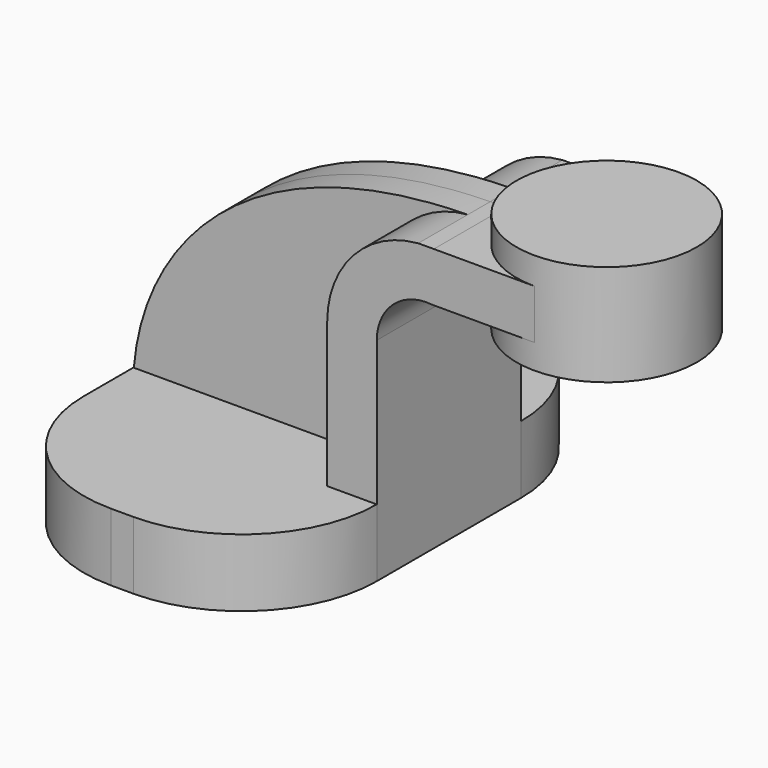
from build123d import *

# Parameters (mm, degrees)
F1_DEPTH = 63.5
F2_DEPTH = 25.4
F3_DEPTH = 7.9375
F5_R     = 38.1


with BuildPart() as f1:
    # F0 (on Front) → F1 (new body, symmetric)
    with BuildSketch(Plane.XZ):
        Polygon((41.275, 9.525), (27.305, 9.525), (-41.1475321427, 9.525), (-41.275, 9.525), (-41.275, -9.525), (41.275, -9.525), align=None)
    extrude(amount=F1_DEPTH, both=True)

    # F0 (on Front) → F2 (join, symmetric)
    with BuildSketch(Plane.XZ):
        with BuildLine():
            Line((27.305, 50.2448773877), (27.305, 9.525))
            Line((27.305, 9.525), (41.275, 9.525))
            Line((41.275, 9.525), (41.275, 50.2448773877))
            ThreePointArc((41.275, 50.2448773877), (45.9090266229, 60.6372063424), (56.7367753904, 64.135))
            Line((56.7367753904, 64.135), (60.325, 64.135))
            Line((60.325, 64.135), (60.325, 78.105))
            Line((60.325, 78.105), (57.3562006129, 78.105))
            add(Edge.make_bspline(
                [(52.937874551, 78.0894598439), (54.3919964318, 78.1126841505), (55.864731429, 78.1180111613), (57.3562006129, 78.105)],
                knots=[117.4190282855, 117.4190282855, 117.4190282855, 117.4190282855, 120.108518673, 120.108518673, 120.108518673, 120.108518673], degree=3))
            ThreePointArc((52.937874551, 78.0894598439), (34.6889220053, 69.1681767162), (27.305, 50.2448773877))
        make_face()
        Polygon((60.325, 78.105), (60.325, 64.135), (85.725, 64.135), (85.725, 71.4375), (85.725, 78.105), align=None)
    extrude(amount=F2_DEPTH, both=True)

    # F0 (on Front) → F3 (join, symmetric)
    with BuildSketch(Plane.XZ):
        with BuildLine():
            Line((-41.1475321427, 9.525), (27.305, 9.525))
            Line((27.305, 9.525), (27.305, 50.2448773877))
            ThreePointArc((27.305, 50.2448773877), (34.6889220053, 69.1681767162), (52.937874551, 78.0894598439))
            add(Edge.make_bspline(
                [(-41.1475321427, 9.525), (-38.4794783387, 42.0413634319), (-10.4626480253, 77.0768671657), (52.937874551, 78.0894598439)],
                knots=[0.1557518826, 0.1557518826, 0.1557518826, 0.1557518826, 117.4190282855, 117.4190282855, 117.4190282855, 117.4190282855], degree=3))
        make_face()
    extrude(amount=F3_DEPTH, both=True)

    # F0 (on Front) → F4 (revolve)
    with BuildSketch(Plane.XZ):
        Polygon((85.725, 71.4375), (85.725, 64.135), (85.725, 57.15), (111.125, 57.15), (111.125, 85.725), (85.725, 85.725), (85.725, 78.105), align=None)
    revolve(axis=Axis((85.725, 0, 71.4375), (0, 0, 1)))

    # F5
    f5_edges = [f1.edges().sort_by_distance(p)[0] for p in [
        (-41.275, -63.5, 0),
        (41.275, -63.5, 0),
        (41.275, 63.5, 0),
        (-41.275, 63.5, 0),
    ]]
    fillet(f5_edges, radius=F5_R)


solid = f1.part
